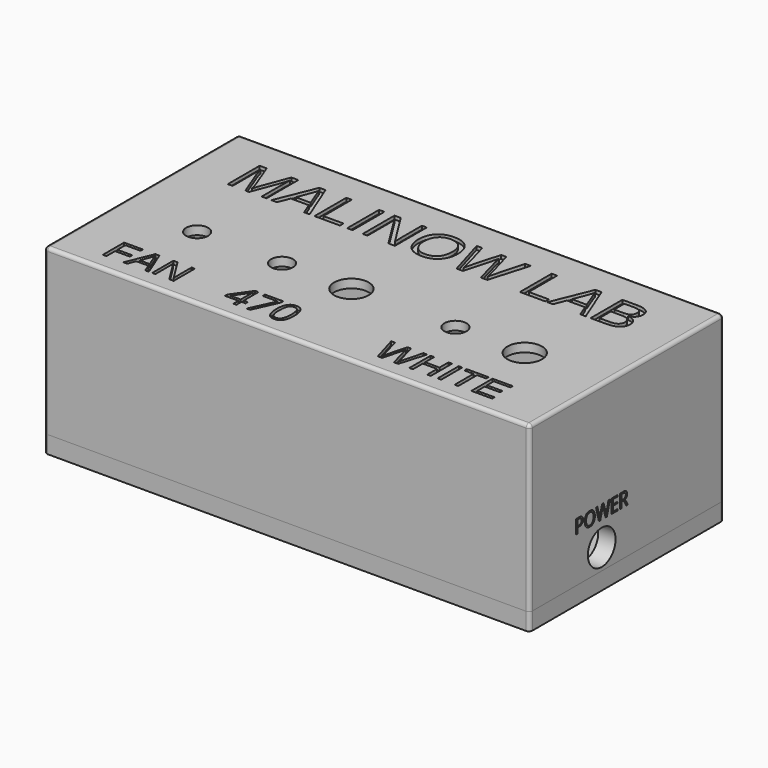
from build123d import *

# Parameters (mm, degrees)
F0_W             = 140
F0_H             = 70
F0_R             = 3.175
F0_R_2           = 5
F1_DEPTH         = 2.5
F2_W             = 140
F2_H             = 70
F2_W_2           = 130
F2_H_2           = 60
F3_DEPTH         = 45
F4_W             = 140
F4_H             = 70
F4_W_2           = 130
F4_H_2           = 60
F5_DEPTH         = 5
F7_D             = 2.4
F7_DEPTH         = 5
F7_CSINK_D       = 4
F7_CSINK_ANGLE   = 90
F7_TIP           = 0.7210327428
F7_2_D           = 2.4
F7_2_DEPTH       = 5
F7_2_CSINK_D     = 4
F7_2_CSINK_ANGLE = 90
F7_2_TIP         = 0.7210327428
F9_D             = 2.9
F9_DEPTH         = 5.2
F9_CBORE_D       = 3.7
F9_CBORE_DEPTH   = 0.2
F9_TIP           = 0.8712478976
F10_R            = 1
F10_2_R          = 1
F13_TEXT_SIZE    = 16.6666666667
F14_DEPTH        = 1
F16_TEXT_SIZE    = 11.1111111111
F17_DEPTH        = 1
F11_R            = 5
F19_DEPTH        = 25
F12_R            = 5
F20_DEPTH        = 25
F21_TEXT_SIZE    = 5.5555555556
F22_DEPTH        = 2
F23_TEXT_SIZE    = 5.5555555556
F24_DEPTH        = 2
F25_R            = 1


# Not quite as in the source:
# - Text() gives the source's letters only with a copy of the font that has no kerning and outlines rounded to 1/6400 em; it was checked with that copy


with BuildPart() as f1:
    # F0 (on Top) → F1 (new body)
    with BuildSketch(Plane.XY):
        with Locations((70, 35)):
            Rectangle(F0_W, F0_H)
        with Locations((22.5, 27)):
            Circle(F0_R, mode=Mode.SUBTRACT)
        with Locations((47, 27)):
            Circle(F0_R, mode=Mode.SUBTRACT)
        with Locations((67, 27)):
            Circle(F0_R_2, mode=Mode.SUBTRACT)
        with Locations((97, 27)):
            Circle(F0_R, mode=Mode.SUBTRACT)
        with Locations((117, 27)):
            Circle(F0_R_2, mode=Mode.SUBTRACT)
    extrude(amount=F1_DEPTH)

    # F2 (on face) → F3 (join)
    with BuildSketch(Plane(origin=(0, 0, 0), x_dir=(1, 0, 0), z_dir=(0, 0, -1))):
        with Locations((70, -35)):
            Rectangle(F2_W, F2_H)
        with Locations((70, -35)):
            Rectangle(F2_W_2, F2_H_2, mode=Mode.SUBTRACT)
    extrude(amount=F3_DEPTH)

    # F7
    with Locations(Plane(origin=(0, 0, -50), x_dir=(1, 0, 0), z_dir=(0, 0, -1))):
        with Locations((2.5, -2.5), (2.5, -67.5), (137.5, -67.5), (137.5, -2.5)):
            CounterSinkHole(F7_D / 2, F7_CSINK_D / 2, depth=F7_DEPTH, counter_sink_angle=F7_CSINK_ANGLE)
            with Locations((0, 0, -(F7_DEPTH + F7_TIP / 2))):  # 118° drill point
                Cone(0, F7_D / 2, F7_TIP, mode=Mode.SUBTRACT)

    # F9
    with Locations(Plane(origin=(0, 0, -45), x_dir=(1, 0, 0), z_dir=(0, 0, -1))):
        with Locations((2.5, -2.5), (2.5, -67.5), (137.5, -67.5), (137.5, -2.5)):
            CounterBoreHole(F9_D / 2, F9_CBORE_D / 2, F9_CBORE_DEPTH, depth=F9_DEPTH)
            with Locations((0, 0, -(F9_DEPTH + F9_TIP / 2))):  # 118° drill point
                Cone(0, F9_D / 2, F9_TIP, mode=Mode.SUBTRACT)

    # F10
    f10_edges = [f1.edges().sort_by_distance(p)[0] for p in [
        (70, 0, 2.5),
        (0, 35, 2.5),
        (70, 70, 2.5),
        (140, 35, 2.5),
        (140, 0, -21.25),
        (0, 0, -21.25),
        (140, 70, -21.25),
        (0, 70, -21.25),
    ]]
    fillet(f10_edges, radius=F10_R)

    # F13 (on face) → F14 (cut)
    with BuildSketch(Plane.XY.offset(2.5)):
        with Locations((11.98046875, 49.5)):
            Text('MALINOW LAB', F13_TEXT_SIZE, font='Arimo', text_align=(TextAlign.LEFT, TextAlign.BOTTOM))
    extrude(amount=-F14_DEPTH, mode=Mode.SUBTRACT)

    # F15: union 

    # F16 (on face) → F17 (cut)
    with BuildSketch(Plane.XY.offset(2.5)):
        with Locations((12, 5)):
            Text('FAN', F16_TEXT_SIZE, font='Arimo', text_align=(TextAlign.LEFT, TextAlign.BOTTOM))
        with Locations((89.9097222222, 5)):
            Text('WHITE', F16_TEXT_SIZE, font='Arimo', text_align=(TextAlign.LEFT, TextAlign.BOTTOM))
        with Locations((46.6840277778, 4.7221066505)):
            Text('470', F16_TEXT_SIZE, font='Open Sans', text_align=(TextAlign.LEFT, TextAlign.BOTTOM))
    extrude(amount=-F17_DEPTH, mode=Mode.SUBTRACT)

    # F11 (on face) → F19 (cut)
    with BuildSketch(Plane(origin=(0, 0, 0), x_dir=(0, -1, 0), z_dir=(-1, 0, 0))):
        with Locations((-20, -39)):
            Circle(F11_R)
        with Locations((-35, -39)):
            Circle(F11_R)
        with Locations((-50, -39)):
            Circle(F11_R)
    extrude(amount=-F19_DEPTH, mode=Mode.SUBTRACT)

    # F12 (on face) → F20 (cut)
    with BuildSketch(Plane.YZ.offset(140)):
        with Locations((26, -39)):
            Circle(F12_R)
    extrude(amount=-F20_DEPTH, mode=Mode.SUBTRACT)

    # F21 (on face) → F22 (cut)
    with BuildSketch(Plane(origin=(0, 0, 0), x_dir=(0, -1, 0), z_dir=(-1, 0, 0))):
        with Locations((-55, -32)):
            Text('FAN   470  WHITE', F21_TEXT_SIZE, font='Open Sans', text_align=(TextAlign.LEFT, TextAlign.BOTTOM))
    extrude(amount=-F22_DEPTH, mode=Mode.SUBTRACT)

    # F23 (on face) → F24 (cut)
    with BuildSketch(Plane.YZ.offset(140)):
        with Locations((16.1983506944, -32)):
            Text('POWER', F23_TEXT_SIZE, font='Open Sans', text_align=(TextAlign.LEFT, TextAlign.BOTTOM))
    extrude(amount=-F24_DEPTH, mode=Mode.SUBTRACT)

    # F25
    f25_edges = [f1.edges().sort_by_distance(p)[0] for p in [
        (5, 5, -22.5),
        (135, 5, -22.5),
        (135, 65, -22.5),
        (5, 65, -22.5),
    ]]
    fillet(f25_edges, radius=F25_R)


with BuildPart() as f5:
    # F4 (on face) → F5 (new body)
    with BuildSketch(Plane(origin=(0, 0, -45), x_dir=(1, 0, 0), z_dir=(0, 0, -1))):
        with Locations((70, -35)):
            Rectangle(F4_W, F4_H)
        with Locations((70, -35)):
            Rectangle(F4_W_2, F4_H_2, mode=Mode.SUBTRACT)
        with Locations((70, -35)):
            Rectangle(F4_W_2, F4_H_2)
    extrude(amount=F5_DEPTH)

    # F7#2
    with Locations(Plane(origin=(0, 0, -50), x_dir=(1, 0, 0), z_dir=(0, 0, -1))):
        with Locations((2.5, -2.5), (2.5, -67.5), (137.5, -67.5), (137.5, -2.5)):
            CounterSinkHole(F7_2_D / 2, F7_2_CSINK_D / 2, depth=F7_2_DEPTH, counter_sink_angle=F7_2_CSINK_ANGLE)
            with Locations((0, 0, -(F7_2_DEPTH + F7_2_TIP / 2))):  # 118° drill point
                Cone(0, F7_2_D / 2, F7_2_TIP, mode=Mode.SUBTRACT)

    # F10#2
    f10_2_edges = [f5.edges().sort_by_distance(p)[0] for p in [
        (0, 70, -47.5),
        (0, 0, -47.5),
        (140, 70, -47.5),
        (140, 0, -47.5),
    ]]
    fillet(f10_2_edges, radius=F10_2_R)


solid = Compound([f1.part, f5.part])
